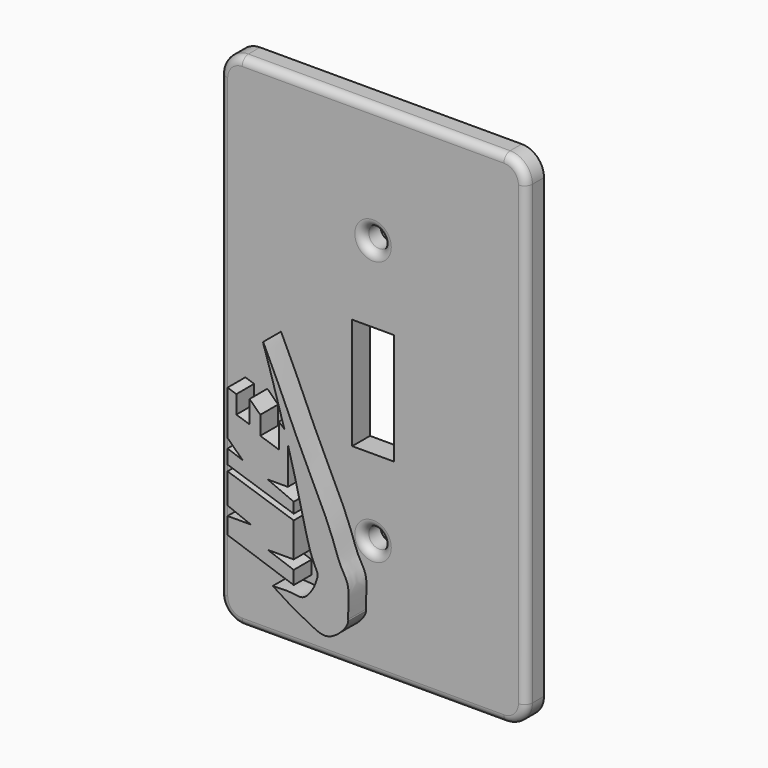
from build123d import *

# Parameters (mm, degrees)
F2_DEPTH     = 5.08
F3_DEPTH     = 5.08
F4_R         = 1.778
F5_R         = 1.778
F6_T         = 2.54
F6_T3_DEPTH  = 10.16
F7_T1_DEPTH  = 17.78
F7_T4_ANGLE  = 90
F7_T6_ANGLE  = 90
F7_T8_ANGLE  = 90
F7_T10_ANGLE = 90


# Not quite as in the source:
# - a fillet or chamfer that OpenCascade refuses, or shapes differently, is made with other operations: its cross-section is extruded or revolved along the edge and cut away or added
# - a shell that OpenCascade refuses in one call is made with other operations: the cavity is built on its own and cut out


with BuildPart() as f2:
    # F1 (on face) → F2 (new body)
    with BuildSketch(Plane.XZ):
        Polygon((-29.1207358241, -36.39671579), (-14.0353180468, -41.5524914861), (-14.0353180468, -38.4972169995), (-19.9549123645, -36.39671579), (-14.0353180468, -36.39671579), (-14.0353180468, -35.0600332022), (-14.0353180468, -32.5776226819), (-29.1207358241, -27.6128016412), (-29.1207358241, -30.4771214724), (-23.7740054727, -32.5776226819), (-29.1207358241, -32.5776226819), align=None)
        Polygon((-29.1207358241, -26.085164398), (-29.1207358241, -27.6128016412), (-14.0353180468, -32.5776226819), align=None)
        Polygon((-29.1207358241, -26.085164398), (-14.0353180468, -32.5776226819), (-14.0353180468, -28.5675749183), (-29.1207358241, -23.6027538776), align=None)
    extrude(amount=F2_DEPTH)


with BuildPart() as f2b:
    # F1 (on face) → F2, piece 2 (new body)
    with BuildSketch(Plane.XZ):
        Polygon((-29.1207358241, -19.0198421478), (-29.1207358241, -22.2660731524), (-14.0353180468, -27.2308941931), (-14.0353180468, -24.8137466562), (-19.9549123645, -22.2660731524), (-15.3720006347, -22.2660731524), (-15.3720006347, -19.0198421478), (-23.9926046991, -19.0198421478), (-29.1207358241, -14.0550211072), (-29.1207358241, -16.9193409383), (-25.6959052529, -20.2351046086), align=None)
        Polygon((-15.3720006347, -19.0198421478), (-29.1207358241, -14.0550211072), (-23.9926046991, -19.0198421478), align=None)
        with BuildLine():
            Line((-29.1207358241, -6.7987442017), (-29.1207358241, -14.0550211072))
            Line((-29.1207358241, -14.0550211072), (-15.3720006347, -19.0198421478))
            Line((-15.3720006347, -19.0198421478), (-15.3720006347, -13.7269175678))
            add(Edge.make_bspline(
                [(-15.3720006347, -13.7269175678), (-15.637888394, -12.7782191771), (-15.9085277985, -11.8278120048), (-16.1803051625, -10.8857762251)],
                knots=[0.3842505291, 0.3842505291, 0.3842505291, 0.3842505291, 0.3977072203, 0.3977072203, 0.3977072203, 0.3977072203], degree=3))
            Line((-16.1803051625, -10.8857762251), (-17.4233510068, -9.829531051))
            Line((-17.4233510068, -9.829531051), (-17.4233510068, -15.4480042413))
            Line((-17.4233510068, -15.4480042413), (-21.6558766836, -14.0550211072))
            Line((-21.6558766836, -14.0550211072), (-21.6558766836, -9.829531051))
            Line((-21.6558766836, -9.829531051), (-24.1050274968, -7.4583757133))
            Line((-24.1050274968, -7.4583757133), (-24.1050274968, -12.5637194561))
            Line((-24.1050274968, -12.5637194561), (-27.1164708465, -11.5726115182))
            Line((-27.1164708465, -11.5726115182), (-27.1164708465, -7.4583757133))
            Line((-27.1164708465, -7.4583757133), (-29.1207358241, -6.7987442017))
        make_face()
        with BuildLine():
            add(Edge.make_bspline(
                [(-15.3720006347, -13.7269175678), (-15.637888394, -12.7782191771), (-15.9085277985, -11.8278120048), (-16.1803051625, -10.8857762251)],
                knots=[0.3842505291, 0.3842505291, 0.3842505291, 0.3842505291, 0.3977072203, 0.3977072203, 0.3977072203, 0.3977072203], degree=3))
            Line((-15.3720006347, -13.7269175678), (-15.3720006347, -11.5726115182))
            Line((-15.3720006347, -11.5726115182), (-16.1803051625, -10.8857762251))
        make_face()
        with BuildLine():
            Line((-15.3720006347, -11.5726115182), (-15.3720006347, -13.7269175678))
            add(Edge.make_bspline(
                [(-18.809184432, -43.27108711), (-17.2052650712, -43.1970243349), (-14.4084211665, -43.0678769313), (-11.6847572425, -43.8896624921), (-9.3937007524, -40.723847522), (-8.8132484367, -38.8262209091), (-8.3460034767, -37.4711265044), (-10.4963241945, -34.3752959777), (-12.3738311652, -24.7044167605), (-14.8694560957, -15.5200170192), (-15.3720006347, -13.7269175678)],
                knots=[0, 0, 0, 0, 0.0549584655, 0.0958341503, 0.1441194546, 0.1813250192, 0.2092854461, 0.2535305673, 0.358816539, 0.3842505291, 0.3842505291, 0.3842505291, 0.3842505291], degree=3))
            add(Edge.make_bspline(
                [(-18.809184432, -43.27108711), (-16.5611162912, -44.7151696718), (-13.4529813666, -46.766729087), (-10.24017934, -48.1024317512), (-5.9782676961, -50.7788277465), (-1.6414231258, -46.0596957731), (-1.5915711613, -44.7150585131)],
                knots=[0, 0, 0, 0, 0.2823165992, 0.4866985275, 0.7211389315, 0.9794325382, 0.9794325382, 0.9794325382, 0.9794325382], degree=3))
            add(Edge.make_bspline(
                [(-1.6232648632, -44.4168113172), (-1.6156949285, -44.5253644232), (-1.604948017, -44.6242237773), (-1.5915711613, -44.7150585131)],
                knots=[0.970591982, 0.970591982, 0.970591982, 0.970591982, 0.9756556469, 0.9756556469, 0.9756556469, 0.9756556469], degree=3))
            add(Edge.make_bspline(
                [(-16.1803051625, -10.8857762251), (-17.9410001087, -4.782848403), (-20.3839984557, 2.9868185818), (-21.7129167385, 6.8213645145), (-14.6292829463, -8.5626845594), (-12.1021656612, -14.6519838589), (-5.4188614427, -27.6154174035), (-3.6243554791, -34.4053902949), (-0.9407860634, -37.5724172841), (-1.7215110815, -43.0079573891), (-1.6232648632, -44.4168113172)],
                knots=[0.3977072203, 0.3977072203, 0.3977072203, 0.3977072203, 0.4848856656, 0.5154744581, 0.6100299667, 0.6880075391, 0.7847527855, 0.8531514045, 0.904873326, 0.970591982, 0.970591982, 0.970591982, 0.970591982], degree=3))
            Line((-16.1803051625, -10.8857762251), (-15.3720006347, -11.5726115182))
        make_face()
        with BuildLine():
            add(Edge.make_bspline(
                [(-1.6232648632, -44.4168113172), (-1.6156949285, -44.5253644232), (-1.604948017, -44.6242237773), (-1.5915711613, -44.7150585131)],
                knots=[0.970591982, 0.970591982, 0.970591982, 0.970591982, 0.9756556469, 0.9756556469, 0.9756556469, 0.9756556469], degree=3))
            add(Edge.make_bspline(
                [(-1.5915711613, -44.7150585131), (-1.5876015378, -44.6079874328), (-1.5977306348, -44.5080759346), (-1.6232648632, -44.4168113172)],
                knots=[0.9794325382, 0.9794325382, 0.9794325382, 0.9794325382, 1, 1, 1, 1], degree=3))
        make_face()
    extrude(amount=F2_DEPTH)


with BuildPart() as f3:
    # F0 (on Front) → F3 (new body)
    with BuildSketch(Plane.XZ):
        with BuildLine():
            Line((34.925, -57.15), (34.925, 0))
            Line((34.925, 0), (4.7625, 0))
            Line((4.7625, 0), (4.7625, -12.7))
            Line((4.7625, -12.7), (0, -12.7))
            Line((0, -12.7), (0, -27.79395))
            ThreePointArc((0, -27.79395), (1.6837980227, -28.4914019773), (2.38125, -30.1752))
            ThreePointArc((2.38125, -30.1752), (1.6837980227, -31.8589980227), (0, -32.55645))
            Line((0, -32.55645), (0, -57.15))
            Line((0, -57.15), (34.925, -57.15))
        make_face()
        with BuildLine():
            Line((4.7625, 0), (34.925, 0))
            Line((34.925, 0), (34.925, 57.15))
            Line((34.925, 57.15), (0, 57.15))
            Line((0, 57.15), (0, 32.54375))
            ThreePointArc((0, 32.54375), (1.6837980227, 31.8462980227), (2.38125, 30.1625))
            ThreePointArc((2.38125, 30.1625), (1.6837980227, 28.4787019773), (0, 27.78125))
            Line((0, 27.78125), (0, 12.7))
            Line((0, 12.7), (4.7625, 12.7))
            Line((4.7625, 12.7), (4.7625, 0))
        make_face()
        with BuildLine():
            Line((-34.925, -57.15), (0, -57.15))
            Line((0, -57.15), (0, -32.55645))
            ThreePointArc((0, -32.55645), (-2.38125, -30.1752), (0, -27.79395))
            Line((0, -27.79395), (0, -12.7))
            Line((0, -12.7), (-4.7625, -12.7))
            Line((-4.7625, -12.7), (-4.7625, 0))
            Line((-4.7625, 0), (-34.925, 0))
            Line((-34.925, 0), (-34.925, -57.15))
        make_face()
        with BuildLine():
            Line((0, 32.54375), (0, 57.15))
            Line((0, 57.15), (-34.925, 57.15))
            Line((-34.925, 57.15), (-34.925, 0))
            Line((-34.925, 0), (-4.7625, 0))
            Line((-4.7625, 0), (-4.7625, 12.7))
            Line((-4.7625, 12.7), (0, 12.7))
            Line((0, 12.7), (0, 27.78125))
            ThreePointArc((0, 27.78125), (-2.38125, 30.1625), (0, 32.54375))
        make_face()
    extrude(amount=-F3_DEPTH)

    # F4
    f4_edges = [f3.edges().sort_by_distance(p)[0] for p in [
        (0, 0, 32.54375),
        (0, 0, -27.79395),
    ]]
    fillet(f4_edges, radius=F4_R)

    # F5
    f5_edges = [f3.edges().sort_by_distance(p)[0] for p in [
        (0, 0, 57.15),
        (34.925, 0, 0),
        (-34.925, 0, 0),
        (0, 0, -57.15),
    ]]
    fillet(f5_edges, radius=F5_R)

    # F6: shell of thickness 2.54, made by hand


with BuildPart() as f6_core1:
    # F6_t2: copy of F3
    add(f3.part)

    # the walls: a layer under each face that stays
    f6_faces = [f6_core1.faces().sort_by_distance(p)[0] for p in [
        (-22.098, 0, -36.9146666667),
        (4.7625, 2.54, 0),
        (0, 2.54, -12.7),
        (-4.7625, 2.54, 0),
        (0, 2.54, 12.7),
        (0, 3.429, 57.15),
        (34.925, 3.429, 0),
        (-34.925, 3.429, 0),
        (0, 3.429, -57.15),
        (0, 3.429, 32.54375),
        (0, 3.429, -27.79395),
    ]]
    thicken(f6_faces, amount=-F6_T, mode=Mode.SUBTRACT)

    # F6_s4 → F6_t3 (cut)
    with BuildSketch(Plane.XZ.offset(-7.62)):
        Polygon((4.7371, 12.6746), (7.3025, 12.7), (7.3025, 15.24), (4.7625, 15.24), align=None)
        Polygon((4.7371, -12.6746), (7.3025, -12.7), (7.3025, -15.24), (4.7625, -15.24), align=None)
        Polygon((-4.7371, -12.6746), (-4.7625, -15.24), (-7.3025, -15.24), (-7.3025, -12.7), align=None)
        Polygon((-4.7371, 12.6746), (-7.3025, 12.7), (-7.3025, 15.24), (-4.7625, 15.24), align=None)
    extrude(amount=F6_T3_DEPTH, mode=Mode.SUBTRACT)


with BuildPart() as f3_1:
    add(f3.part)

    # what is left inside the walls is the cavity
    f6_cavity = [f6_core1.part.solids().sort_by_distance(p)[0] for p in [
        (0, 2.5654, -18.203333),
    ]]
    add(f6_cavity, mode=Mode.SUBTRACT)

    # F7: fillet of radius 5.08 on 4 edges, made by hand

    # F7_s2 → F7_t1 (cut)
    with BuildSketch(Plane.XZ.offset(-17.78)):
        with BuildLine():
            ThreePointArc((29.845, 57.15), (33.4371024484, 55.6621024484), (34.925, 52.07))
            Line((34.925, 52.07), (34.925, 57.15))
            Line((34.925, 57.15), (29.845, 57.15))
        make_face()
        with BuildLine():
            ThreePointArc((34.925, -52.07), (33.4371024484, -55.6621024484), (29.845, -57.15))
            Line((29.845, -57.15), (34.925, -57.15))
            Line((34.925, -57.15), (34.925, -52.07))
        make_face()
        with BuildLine():
            ThreePointArc((-29.845, 57.15), (-33.4371024484, 55.6621024484), (-34.925, 52.07))
            Line((-34.925, 52.07), (-34.925, 57.15))
            Line((-34.925, 57.15), (-29.845, 57.15))
        make_face()
        with BuildLine():
            ThreePointArc((-34.925, -52.07), (-33.4371024484, -55.6621024484), (-29.845, -57.15))
            Line((-29.845, -57.15), (-34.925, -57.15))
            Line((-34.925, -57.15), (-34.925, -52.07))
        make_face()
    extrude(amount=F7_T1_DEPTH, mode=Mode.SUBTRACT)

    # F7_s3 → F7_t4 (revolve, cut)
    with BuildSketch(Plane.XY.offset(-52.07)):
        with BuildLine():
            ThreePointArc((-33.147, 0), (-34.4042358569, 0.5207641431), (-34.925, 1.778))
            Line((-34.925, 1.778), (-34.925, 0))
            Line((-34.925, 0), (-33.147, 0))
        make_face()
    revolve(axis=Axis((-29.845, 0, -52.07), (0, -1, 0)), revolution_arc=F7_T4_ANGLE, mode=Mode.SUBTRACT)

    # F7_s5 → F7_t6 (revolve, cut)
    with BuildSketch(Plane.YZ.offset(-29.845)):
        with BuildLine():
            ThreePointArc((0, 55.372), (0.5207641431, 56.6292358569), (1.778, 57.15))
            Line((1.778, 57.15), (0, 57.15))
            Line((0, 57.15), (0, 55.372))
        make_face()
    revolve(axis=Axis((-29.845, 0, 52.07), (0, -1, 0)), revolution_arc=F7_T6_ANGLE, mode=Mode.SUBTRACT)

    # F7_s7 → F7_t8 (revolve, cut)
    with BuildSketch(Plane.YZ.offset(29.845)):
        with BuildLine():
            ThreePointArc((0, -55.372), (0.5207641431, -56.6292358569), (1.778, -57.15))
            Line((1.778, -57.15), (0, -57.15))
            Line((0, -57.15), (0, -55.372))
        make_face()
    revolve(axis=Axis((29.845, 0, -52.07), (0, -1, 0)), revolution_arc=F7_T8_ANGLE, mode=Mode.SUBTRACT)

    # F7_s9 → F7_t10 (revolve, cut)
    with BuildSketch(Plane.XY.offset(52.07)):
        with BuildLine():
            ThreePointArc((33.147, 0), (34.4042358569, 0.5207641431), (34.925, 1.778))
            Line((34.925, 1.778), (34.925, 0))
            Line((34.925, 0), (33.147, 0))
        make_face()
    revolve(axis=Axis((29.845, 0, 52.07), (0, -1, 0)), revolution_arc=F7_T10_ANGLE, mode=Mode.SUBTRACT)


solid = Compound([f2.part, f2b.part, f3_1.part])
